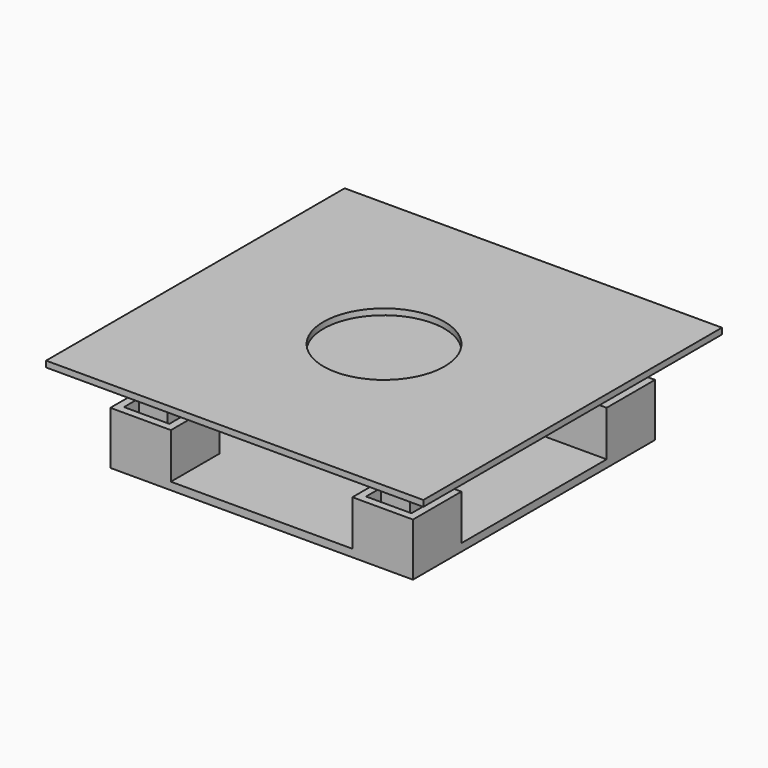
from build123d import *

# Parameters (mm, degrees)
F0_W      = 20
F0_H      = 20
F1_DEPTH  = 0.5
F2_W      = 4
F2_H      = 4
F2_W_2    = 3
F2_H_2    = 3
F3_DEPTH  = 3
F2_W_3    = 1.9
F2_H_3    = 1.9
F4_DEPTH  = 6
F5_W      = 24.9357379507
F5_H      = 24.6656327508
F5_W_2    = 1.9
F5_H_2    = 1.9
F6_DEPTH  = 0.4
F7_R      = 4
F8_DEPTH  = 25
F9_R      = 6.1663142181
F10_DEPTH = 2.5
F11_W     = 7.5
F11_H     = 7.5
F12_DEPTH = 2
F13_W     = 4.95
F13_H     = 0.875
F14_DEPTH = 1
F15_R     = 1.5
F16_W     = 15
F16_H     = 2.25
F17_DEPTH = 2.5
F18_W     = 1.6371783766
F18_H     = 0.75
F19_DEPTH = 1
F20_W     = 3
F20_H     = 3
F21_DEPTH = 1.5
F22_SIZE2 = 1.24999
F22_SIZE  = 1.49999


# Not quite as in the source:
# - a fillet or chamfer is up to 0.001 mm smaller than in the source, because OpenCascade refuses the exact size
# - a feature names something its author has since deleted; it is built from what else it names


with BuildPart() as f1:
    # F0 (on Top) → F1 (new body)
    with BuildSketch(Plane.XY):
        with Locations((10, 10)):
            Rectangle(F0_W, F0_H)
    extrude(amount=F1_DEPTH)

    # F2 (on face) → F3 (join)
    with BuildSketch(Plane.XY.offset(0.5)):
        with Locations((18, 18)):
            Rectangle(F2_W, F2_H)
        with Locations((18, 18)):
            Rectangle(F2_W_2, F2_H_2, mode=Mode.SUBTRACT)
        with Locations((2, 18)):
            Rectangle(F2_W, F2_H)
        with Locations((2, 18)):
            Rectangle(F2_W_2, F2_H_2, mode=Mode.SUBTRACT)
        with Locations((2, 2)):
            Rectangle(F2_W, F2_H)
        with Locations((2, 2)):
            Rectangle(F2_W_2, F2_H_2, mode=Mode.SUBTRACT)
        with Locations((18, 2)):
            Rectangle(F2_W, F2_H)
        with Locations((18, 2)):
            Rectangle(F2_W_2, F2_H_2, mode=Mode.SUBTRACT)
    extrude(amount=F3_DEPTH)

    # F11 (on face) → F12 (join)
    with BuildSketch(Plane.XY.offset(0.5)):
        with Locations((10, 10)):
            Rectangle(F11_W, F11_H)
    extrude(amount=F12_DEPTH)

    # F13 (on face) → F14 (join)
    with BuildSketch(Plane.XY.offset(2.5)):
        Polygon((12.475, 7.125), (12.475, 6.25), (13.75, 6.25), (13.75, 13.75), (12.475, 13.75), align=None)
        with Locations((10, 6.6875)):
            Rectangle(F13_W, F13_H)
        Polygon((6.25, 6.25), (7.525, 6.25), (7.525, 7.125), (7.525, 13.75), (6.25, 13.75), align=None)
    extrude(amount=F14_DEPTH)

    # F15
    f15_edges = [f1.edges().sort_by_distance(p)[0] for p in [
        (6.25, 13.75, 2),
        (13.75, 13.75, 2),
        (13.75, 6.25, 2),
        (6.25, 6.25, 2),
    ]]
    fillet(f15_edges, radius=F15_R)


with BuildPart() as f4:
    # F2 (on face) → F4 (new body)
    with BuildSketch(Plane.XY.offset(0.5)):
        with Locations((2, 18)):
            Rectangle(F2_W_3, F2_H_3)
    extrude(amount=F4_DEPTH)



with BuildPart() as f4b:
    # F2 (on face) → F4, piece 2 (new body)
    with BuildSketch(Plane.XY.offset(0.5)):
        with Locations((18, 18)):
            Rectangle(F2_W_3, F2_H_3)
    extrude(amount=F4_DEPTH)


with BuildPart() as f4c:
    # F2 (on face) → F4, piece 3 (new body)
    with BuildSketch(Plane.XY.offset(0.5)):
        with Locations((18, 2)):
            Rectangle(F2_W_3, F2_H_3)
    extrude(amount=F4_DEPTH)


with BuildPart() as f4d:
    # F2 (on face) → F4, piece 4 (new body)
    with BuildSketch(Plane.XY.offset(0.5)):
        with Locations((2, 2)):
            Rectangle(F2_W_3, F2_H_3)
    extrude(amount=F4_DEPTH)


with BuildPart() as f4_1:
    add(f4.part)

    add(f4b.part)  # F6 merges F4b

    add(f4c.part)  # F6 merges F4c

    add(f4d.part)  # F6 merges F4d
    # F5 (on face) → F6 (join)
    with BuildSketch(Plane.XY.offset(6.5)):
        with Locations((10.1846862817, 9.8774891812)):
            Rectangle(F5_W, F5_H)
        with Locations((18, 18)):
            Rectangle(F5_W_2, F5_H_2, mode=Mode.SUBTRACT)
    extrude(amount=-F6_DEPTH)

    # F7 (on face) → F8 (cut)
    with BuildSketch(Plane.XY.offset(6.5)):
        with Locations((10.1846862817, 9.8774891812)):
            Circle(F7_R)
    extrude(amount=-F8_DEPTH, mode=Mode.SUBTRACT)

    # F9 (on face) → F10 (join)
    with BuildSketch(Plane(origin=(0, 0, 6.1), x_dir=(1, 0, 0), z_dir=(0, 0, -1))):
        with Locations((10.1846862817, -9.8774891812)):
            Circle(F9_R)
        with BuildLine():
            ThreePointArc((11.1682663292, -15.369970548), (10.571768696, -15.4439017135), (9.970779517, -15.4532425089))
            ThreePointArc((9.970779517, -15.4532425089), (5.0496141216, -7.6944144723), (14.0514253314, -5.8546654968))
            ThreePointArc((14.0514253314, -5.8546654968), (14.4219337589, -6.2469912689), (14.7528122455, -6.6732722014))
            ThreePointArc((14.7528122455, -6.6732722014), (15.066029035, -7.1742921482), (15.3245095344, -7.7056240368))
            ThreePointArc((15.3245095344, -7.7056240368), (15.6534269731, -8.7694925543), (15.7645412327, -9.8774891812))
            ThreePointArc((15.7645412327, -9.8774891812), (15.6534269731, -10.9854858082), (15.3245095344, -12.0493543256))
            ThreePointArc((15.3245095344, -12.0493543256), (13.6675931163, -14.2368631336), (11.1682663292, -15.369970548))
        make_face(mode=Mode.SUBTRACT)
        with BuildLine():
            ThreePointArc((15.7645412327, -9.8774891812), (15.6534269731, -8.7694925543), (15.3245095344, -7.7056240368))
            Line((15.3245095344, -7.7056240368), (15.3245095344, -12.0493543256))
            ThreePointArc((15.3245095344, -12.0493543256), (15.6534269731, -10.9854858082), (15.7645412327, -9.8774891812))
        make_face()
        with BuildLine():
            Line((10.7477184775, -14.5274891812), (10.1846862817, -14.5274891812))
            Line((10.1846862817, -14.5274891812), (9.970779517, -15.4532425089))
            ThreePointArc((9.970779517, -15.4532425089), (10.571768696, -15.4439017135), (11.1682663292, -15.369970548))
            Line((11.1682663292, -15.369970548), (10.7477184775, -14.5274891812))
        make_face()
        with BuildLine():
            Line((13.5860960398, -6.6970156854), (13.7467929422, -6.8885267962))
            Line((13.7467929422, -6.8885267962), (13.9074898446, -7.080037907))
            Line((13.9074898446, -7.080037907), (14.7528122455, -6.6732722014))
            ThreePointArc((14.7528122455, -6.6732722014), (14.4219337589, -6.2469912689), (14.0514253314, -5.8546654968))
            Line((14.0514253314, -5.8546654968), (13.5860960398, -6.6970156854))
        make_face()
    extrude(amount=F10_DEPTH)

    # F16 (on face) → F17 (cut, through all)
    with BuildSketch(Plane(origin=(0, 0, 3.6), x_dir=(1, 0, 0), z_dir=(0, 0, -1))):
        with Locations((10.1846862817, -9.8774891812)):
            Rectangle(F16_W, F16_H)
    extrude(amount=-F17_DEPTH, mode=Mode.SUBTRACT)


with BuildPart() as f19:
    # F18 (on face) → F19 (new body)
    with BuildSketch(Plane(origin=(0, 0, 6.1), x_dir=(1, 0, 0), z_dir=(0, 0, -1))):
        with BuildLine():
            Line((10.1846862817, -9.8774891812), (14.1846862817, -9.8774891812))
            ThreePointArc((14.1846862817, -9.8774891812), (14.1669113912, -9.5008153472), (14.1137446931, -9.1274891812))
            Line((14.1137446931, -9.1274891812), (6.2556278703, -9.1274891812))
            ThreePointArc((6.2556278703, -9.1274891812), (6.2024611722, -9.5008153472), (6.1846862817, -9.8774891812))
            Line((6.1846862817, -9.8774891812), (10.1846862817, -9.8774891812))
        make_face()
        with BuildLine():
            Line((16.0475079051, -9.8774891812), (14.1846862817, -9.8774891812))
            ThreePointArc((14.1846862817, -9.8774891812), (14.1669113912, -10.2541630153), (14.1137446931, -10.6274891812))
            Line((14.1137446931, -10.6274891812), (16.0475079051, -10.6274891812))
            Line((16.0475079051, -10.6274891812), (16.0475079051, -9.8774891812))
        make_face()
        with BuildLine():
            ThreePointArc((14.1137446931, -10.6274891812), (14.1669113912, -10.2541630153), (14.1846862817, -9.8774891812))
            Line((14.1846862817, -9.8774891812), (10.1846862817, -9.8774891812))
            Line((10.1846862817, -9.8774891812), (6.1846862817, -9.8774891812))
            ThreePointArc((6.1846862817, -9.8774891812), (6.2024611722, -10.2541630153), (6.2556278703, -10.6274891812))
            Line((6.2556278703, -10.6274891812), (14.1137446931, -10.6274891812))
        make_face()
        with BuildLine():
            ThreePointArc((14.1137446931, -9.1274891812), (14.1669113912, -9.5008153472), (14.1846862817, -9.8774891812))
            Line((14.1846862817, -9.8774891812), (16.0475079051, -9.8774891812))
            Line((16.0475079051, -9.8774891812), (16.0475079051, -9.1274891812))
            Line((16.0475079051, -9.1274891812), (14.1137446931, -9.1274891812))
        make_face()
        with BuildLine():
            Line((6.2556278703, -9.1274891812), (14.1137446931, -9.1274891812))
            ThreePointArc((14.1137446931, -9.1274891812), (10.1846862817, -5.8774891812), (6.2556278703, -9.1274891812))
        make_face()
        with BuildLine():
            ThreePointArc((6.2556278703, -10.6274891812), (10.1846862817, -13.8774891812), (14.1137446931, -10.6274891812))
            Line((14.1137446931, -10.6274891812), (6.2556278703, -10.6274891812))
        make_face()
        with Locations((16.8660970934, -9.5024891812)):
            Rectangle(F18_W, F18_H)
        with Locations((16.8660970934, -10.2524891812)):
            Rectangle(F18_W, F18_H)
        with BuildLine():
            ThreePointArc((6.1846862817, -9.8774891812), (6.2024611722, -9.5008153472), (6.2556278703, -9.1274891812))
            Line((6.2556278703, -9.1274891812), (4.3218646583, -9.1274891812))
            Line((4.3218646583, -9.1274891812), (4.3218646583, -9.8774891812))
            Line((4.3218646583, -9.8774891812), (6.1846862817, -9.8774891812))
        make_face()
        Polygon((16.0475079051, -8.3041858837), (16.0475079051, -9.1274891812), (17.6846862817, -9.1274891812), align=None)
        with BuildLine():
            Line((4.3218646583, -10.6274891812), (6.2556278703, -10.6274891812))
            ThreePointArc((6.2556278703, -10.6274891812), (6.2024611722, -10.2541630153), (6.1846862817, -9.8774891812))
            Line((6.1846862817, -9.8774891812), (4.3218646583, -9.8774891812))
            Line((4.3218646583, -9.8774891812), (4.3218646583, -10.6274891812))
        make_face()
        Polygon((17.6846862817, -10.6274891812), (16.0475079051, -10.6274891812), (16.0475079051, -11.4507924787), align=None)
        with Locations((3.50327547, -9.5024891812)):
            Rectangle(F18_W, F18_H)
        Polygon((2.6846862817, -9.1274891812), (4.3218646583, -9.1274891812), (4.3218646583, -8.3041858837), align=None)
        Polygon((4.3218646583, -11.4507924787), (4.3218646583, -10.6274891812), (2.6846862817, -10.6274891812), align=None)
        with Locations((3.50327547, -10.2524891812)):
            Rectangle(F18_W, F18_H)
    extrude(amount=F19_DEPTH)

    # F20 (on face) → F21 (join)
    with BuildSketch(Plane(origin=(0, 0, 5.1), x_dir=(1, 0, 0), z_dir=(0, 0, -1))):
        with Locations((10.1846862817, -9.8774891812)):
            Rectangle(F20_W, F20_H)
    extrude(amount=F21_DEPTH)

    # F22 (size 1.5 and 1.25 in the source; OpenCascade refuses exactly that, so slightly less here)
    f22_edges = [f19.edges().sort_by_distance(p)[0] for p in [
        (10.184686, 8.377489, 3.6),
        (8.684686, 9.877489, 3.6),
        (10.184686, 11.377489, 3.6),
        (11.684686, 9.877489, 3.6),
    ]]
    chamfer(f22_edges, length=F22_SIZE, length2=F22_SIZE2)


solid = Compound([f1.part, f4_1.part, f19.part])
